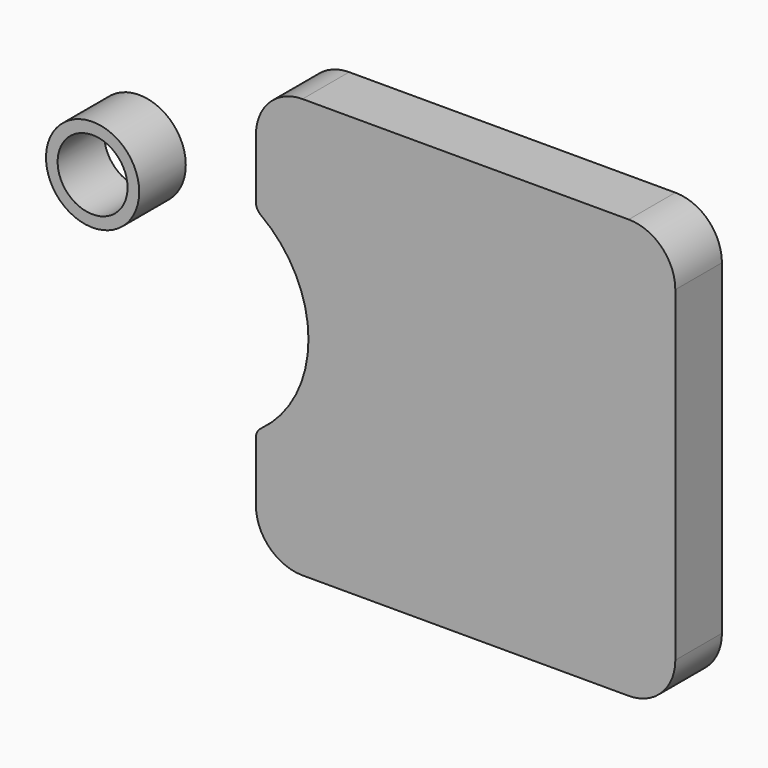
from build123d import *

# Parameters (mm, degrees)
F1_DEPTH = 25
F2_R     = 20
F2_R_2   = 15
F3_DEPTH = 25
F4_R     = 5


with BuildPart() as f1:
    # F0 (on Front) → F1 (new body)
    with BuildSketch(Plane.XZ):
        with BuildLine():
            Line((70, 90), (-70, 90))
            ThreePointArc((-70, 90), (-84.1421356237, 84.1421356237), (-90, 70))
            Line((-90, 70), (-90, 41.7921018494))
            ThreePointArc((-90, 41.7921018494), (-67.4485012889, 0), (-90, -41.7921018494))
            Line((-90, -41.7921018494), (-90, -70))
            ThreePointArc((-90, -70), (-84.1421356237, -84.1421356237), (-70, -90))
            Line((-70, -90), (70, -90))
            ThreePointArc((70, -90), (84.1421356237, -84.1421356237), (90, -70))
            Line((90, -70), (90, 70))
            ThreePointArc((90, 70), (84.1421356237, 84.1421356237), (70, 90))
        make_face()
    extrude(amount=F1_DEPTH)

    # F4
    f4_edges = [f1.edges().sort_by_distance(p)[0] for p in [
        (-90, -12.5, -41.792102),
        (-90, -12.5, 41.792102),
    ]]
    fillet(f4_edges, radius=F4_R)


with BuildPart() as f3:
    # F2 (on Front) → F3 (new body)
    with BuildSketch(Plane.XZ):
        with Locations((-160.1076126099, 32.092448324)):
            Circle(F2_R)
        with Locations((-160.1076126099, 32.092448324)):
            Circle(F2_R_2, mode=Mode.SUBTRACT)
    extrude(amount=F3_DEPTH)


solid = Compound([f1.part, f3.part])
